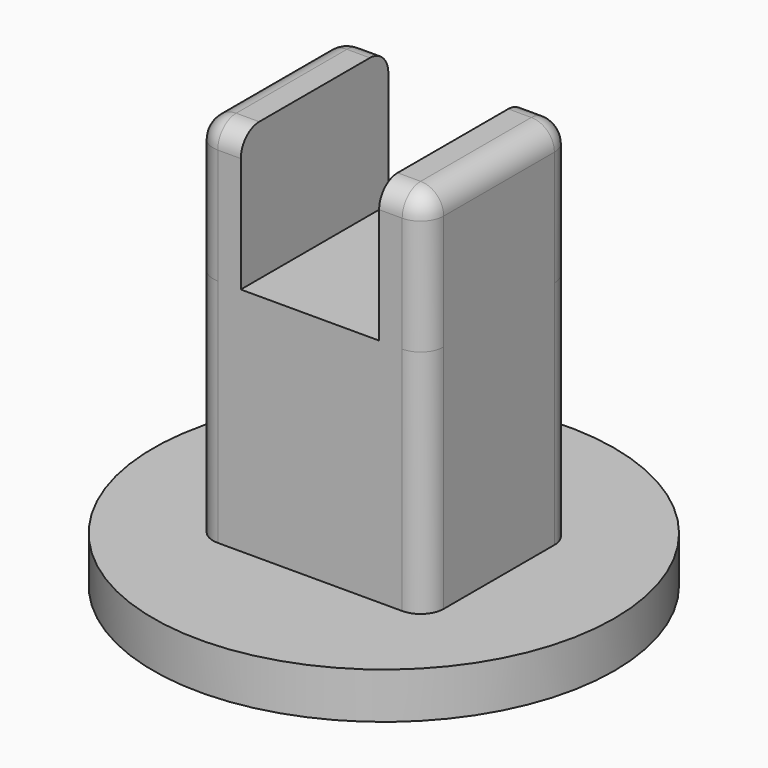
from build123d import *

# Parameters (mm, degrees)
F1_DEPTH  = 76.2
F2_R      = 63.5
F3_DEPTH  = 12.7
F5_W      = 38.1
F5_H      = 38.1
F5_H_2    = 63.5
F6_DEPTH  = 12.7
F7_DEPTH  = 6.35
F8_DEPTH  = 6.35
F9_R      = 6.35
F10_W     = 38.1
F10_H     = 38.1
F11_DEPTH = 12.7
F12_DEPTH = 6.35
F13_DEPTH = 6.35
F14_R     = 6.35


with BuildPart() as f1:
    # F0 (on Top) → F1 (new body)
    with BuildSketch(Plane.XY):
        with BuildLine():
            Line((-74.277333, 16.310153), (-125.077333, 16.310153))
            ThreePointArc((-125.077333, 16.310153), (-129.567461, 14.450281), (-131.427333, 9.960153))
            Line((-131.427333, 9.960153), (-131.427333, -28.139847))
            ThreePointArc((-131.427333, -28.139847), (-129.567461, -32.629975), (-125.077333, -34.489847))
            Line((-125.077333, -34.489847), (-74.277333, -34.489847))
            ThreePointArc((-74.277333, -34.489847), (-69.787205, -32.629975), (-67.927333, -28.139847))
            Line((-67.927333, -28.139847), (-67.927333, 9.960153))
            ThreePointArc((-67.927333, 9.960153), (-69.787205, 14.450281), (-74.277333, 16.310153))
        make_face()
    extrude(amount=F1_DEPTH)

    # F2 (on Top) → F3 (join)
    with BuildSketch(Plane.XY):
        with Locations((-99.983416, -8.677237)):
            Circle(F2_R)
    extrude(amount=F3_DEPTH)

    # F5 (on face) → F6 (join)
    with BuildSketch(Plane(origin=(-131.427333, 0, 0), x_dir=(0, -1, 0), z_dir=(-1, 0, 0))):
        with Locations((9.089847, 95.25)):
            Rectangle(F5_W, F5_H)
        with Locations((9.089847, 44.45)):
            Rectangle(F5_W, F5_H_2)
    extrude(amount=-F6_DEPTH)

    # F7 (add): a face of the model
    f7_faces = [f1.faces().sort_by_distance(p)[0] for p in [
        (-125.077333, 9.960153, 95.25),
    ]]
    extrude(f7_faces, amount=F7_DEPTH)

    # F8 (add): a face of the model
    f8_faces = [f1.faces().sort_by_distance(p)[0] for p in [
        (-125.077333, -28.139847, 95.25),
    ]]
    extrude(f8_faces, amount=F8_DEPTH)

    # F9
    f9_edges = [f1.edges().sort_by_distance(p)[0] for p in [
        (-125.077333, -34.489847, 114.3),
        (-125.077333, 16.310153, 114.3),
    ]]
    fillet(f9_edges, radius=F9_R)

    # F10 (on face) → F11 (join)
    with BuildSketch(Plane.YZ.offset(-67.927333)):
        with Locations((-9.089847, 95.25)):
            Rectangle(F10_W, F10_H)
    extrude(amount=-F11_DEPTH)

    # F12 (add): a face of the model
    f12_faces = [f1.faces().sort_by_distance(p)[0] for p in [
        (-74.277333, 9.960153, 95.25),
    ]]
    extrude(f12_faces, amount=F12_DEPTH)

    # F13 (add): a face of the model
    f13_faces = [f1.faces().sort_by_distance(p)[0] for p in [
        (-74.277333, -28.139847, 95.25),
    ]]
    extrude(f13_faces, amount=F13_DEPTH)

    # F14
    f14_edges = [f1.edges().sort_by_distance(p)[0] for p in [
        (-131.427333, -34.489847, 92.075),
        (-67.927333, -34.489847, 95.25),
        (-67.927333, 16.310153, 95.25),
        (-67.927333, -9.089847, 114.3),
        (-74.277333, -34.489847, 114.3),
        (-74.277333, 16.310153, 114.3),
    ]]
    fillet(f14_edges, radius=F14_R)


solid = f1.part
